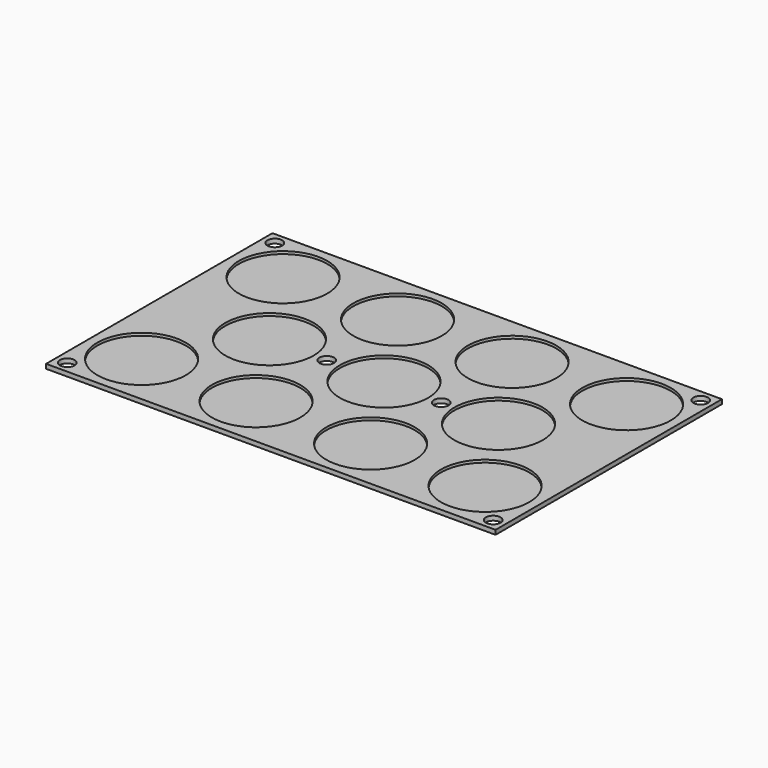
from build123d import *

# Parameters (mm, degrees)
F0_W     = 152.5
F0_H     = 96
F0_R     = 15
F1_DEPTH = 0.9
F2_DEPTH = 0.6
F3_R     = 2.5
F4_DEPTH = 1.501


# Not quite as in the source:
# - a feature names something its author has since deleted; it is built from what else it names


with BuildPart() as f1:
    # F0 (on Top) → F1 (new body)
    with BuildSketch(Plane.XY):
        Rectangle(F0_W, F0_H)
        with Locations((-58.25, -30)):
            Circle(F0_R, mode=Mode.SUBTRACT)
        with Locations((-19.4, -30)):
            Circle(F0_R, mode=Mode.SUBTRACT)
        with Locations((19.45, -30)):
            Circle(F0_R, mode=Mode.SUBTRACT)
        with Locations((58.3, -30)):
            Circle(F0_R, mode=Mode.SUBTRACT)
        with Locations((-38.85, 0)):
            Circle(F0_R, mode=Mode.SUBTRACT)
        with Locations((-58.25, 30)):
            Circle(F0_R, mode=Mode.SUBTRACT)
        with Locations((-19.4, 30)):
            Circle(F0_R, mode=Mode.SUBTRACT)
        Circle(F0_R, mode=Mode.SUBTRACT)
        with Locations((38.85, 0)):
            Circle(F0_R, mode=Mode.SUBTRACT)
        with Locations((19.45, 30)):
            Circle(F0_R, mode=Mode.SUBTRACT)
        with Locations((58.3, 30)):
            Circle(F0_R, mode=Mode.SUBTRACT)
    extrude(amount=F1_DEPTH)

    # F0 (on Top) → F2 (join)
    with BuildSketch(Plane.XY):
        Rectangle(F0_W, F0_H)
        with Locations((-58.25, -30)):
            Circle(F0_R, mode=Mode.SUBTRACT)
        with Locations((-19.4, -30)):
            Circle(F0_R, mode=Mode.SUBTRACT)
        with Locations((19.45, -30)):
            Circle(F0_R, mode=Mode.SUBTRACT)
        with Locations((58.3, -30)):
            Circle(F0_R, mode=Mode.SUBTRACT)
        with Locations((-38.85, 0)):
            Circle(F0_R, mode=Mode.SUBTRACT)
        with Locations((-58.25, 30)):
            Circle(F0_R, mode=Mode.SUBTRACT)
        with Locations((-19.4, 30)):
            Circle(F0_R, mode=Mode.SUBTRACT)
        Circle(F0_R, mode=Mode.SUBTRACT)
        with Locations((38.85, 0)):
            Circle(F0_R, mode=Mode.SUBTRACT)
        with Locations((19.45, 30)):
            Circle(F0_R, mode=Mode.SUBTRACT)
        with Locations((58.3, 30)):
            Circle(F0_R, mode=Mode.SUBTRACT)
        with Locations((-58.25, -30)):
            Circle(F0_R)
        with Locations((-38.85, 0)):
            Circle(F0_R)
        with Locations((-58.25, 30)):
            Circle(F0_R)
        with Locations((-19.4, 30)):
            Circle(F0_R)
        with Locations((19.45, 30)):
            Circle(F0_R)
        Circle(F0_R)
        with Locations((38.85, 0)):
            Circle(F0_R)
        with Locations((19.45, -30)):
            Circle(F0_R)
        with Locations((58.3, -30)):
            Circle(F0_R)
        with Locations((58.3, 30)):
            Circle(F0_R)
        with Locations((-19.4, -30)):
            Circle(F0_R)
    extrude(amount=-F2_DEPTH)

    # F3 (on face) → F4 (cut, through all)
    with BuildSketch(Plane.XY.offset(0.9)):
        with Locations((-72.25, 44)):
            Circle(F3_R)
        with Locations((72.25, 44)):
            Circle(F3_R)
        with Locations((-72.25, -44)):
            Circle(F3_R)
        with Locations((72.25, -44)):
            Circle(F3_R)
        with Locations((-19.425, 0)):
            Circle(F3_R)
        with Locations((19.425, 0)):
            Circle(F3_R)
    extrude(amount=-F4_DEPTH, mode=Mode.SUBTRACT)


solid = f1.part
